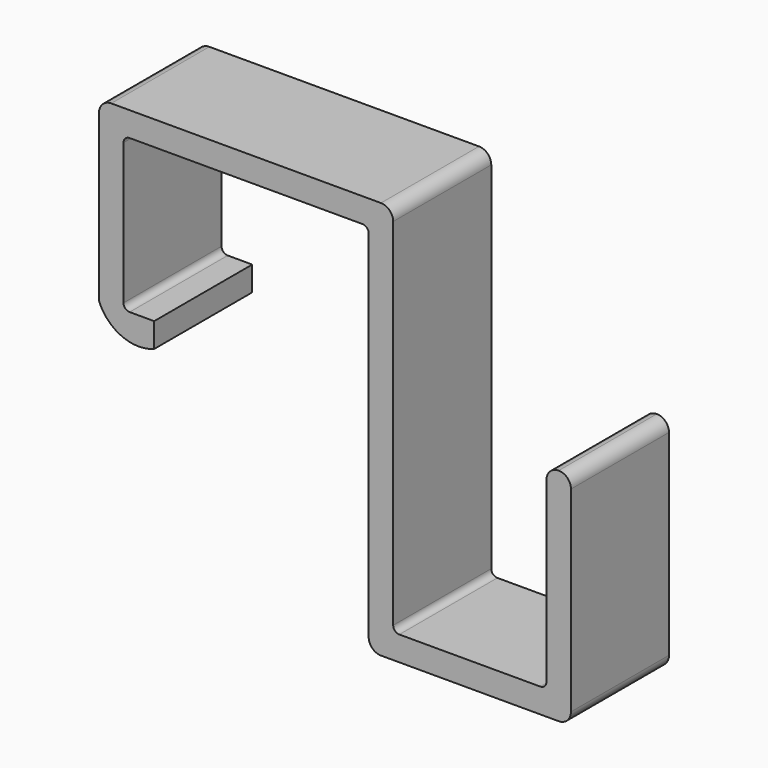
from build123d import *

# Parameters (mm, degrees)
F1_DEPTH = 20
F2_R     = 1
F3_R     = 1.99999


# Not quite as in the source:
# - a fillet or chamfer is up to 0.001 mm smaller than in the source, because OpenCascade refuses the exact size


with BuildPart() as f1:
    # F0 (on Front) → F1 (new body)
    with BuildSketch(Plane.XZ):
        Polygon((-24, 29), (-24, 0), (-20, 0), (-20, 25), (20, 25), (20, -36), (53, -36), (53, 0), (49, 0), (49, -32), (24, -32), (24, 29), align=None)
        with BuildLine():
            Line((-20, 0), (-24, 0))
            ThreePointArc((-24, 0), (-20.3284271247, -3.8639610307), (-15, -4))
            Line((-15, -4), (-15, 0))
            Line((-15, 0), (-20, 0))
        make_face()
    extrude(amount=F1_DEPTH)

    # F2
    f2_edges = [f1.edges().sort_by_distance(p)[0] for p in [
        (-20, -10, 0),
        (-20, -10, 25),
        (20, -10, 25),
        (24, -10, -32),
        (49, -10, -32),
    ]]
    fillet(f2_edges, radius=F2_R)

    # F3 (radius 2 in the source; OpenCascade refuses exactly that, so slightly less here)
    f3_edges = [f1.edges().sort_by_distance(p)[0] for p in [
        (-24, -10, 29),
        (24, -10, 29),
        (20, -10, -36),
        (53, -10, -36),
        (49, -10, 0),
        (53, -10, 0),
    ]]
    fillet(f3_edges, radius=F3_R)


solid = f1.part
